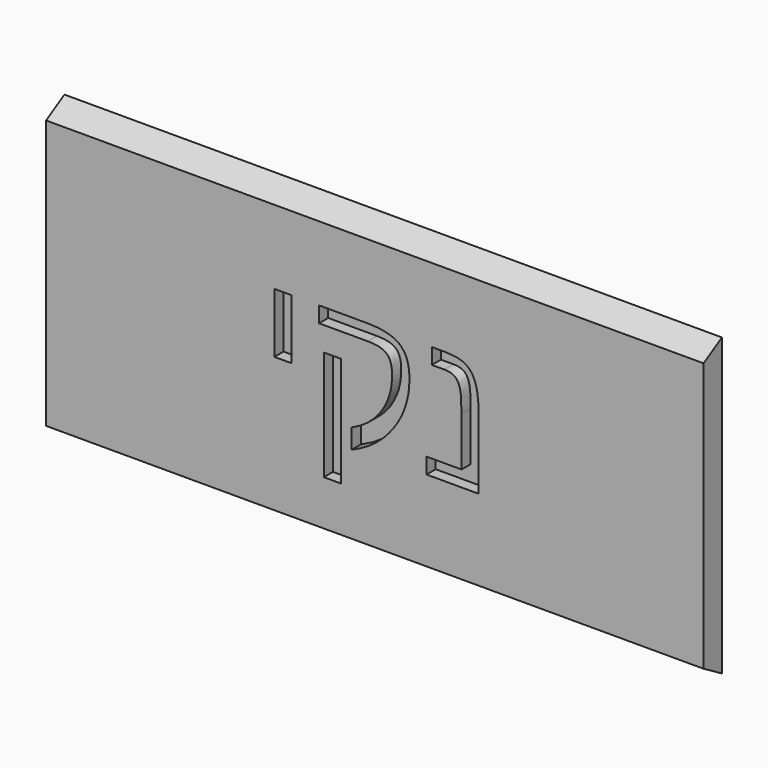
from build123d import *

# Parameters (mm, degrees)
F1_DEPTH     = 36
F2_TEXT_SIZE = 20.8333333333
F3_DEPTH     = 1.3


# Not quite as in the source:
# - Text() gives the source's letters only with a copy of the font that has no kerning and outlines rounded to 1/6400 em; it was checked with that copy


with BuildPart() as f1:
    # F0 (on Right) → F1 (new body, symmetric)
    with BuildSketch(Plane.YZ):
        Polygon((1.2569191167, -16.1964185536), (1.257158001, 16.1968544126), (-1.2568556704, 14.7234033793), (-1.2568556704, -14.7232851014), align=None)
    extrude(amount=F1_DEPTH, both=True)

    # F2 (on Front) → F3 (cut)
    with BuildSketch(Plane.XZ):
        with Locations((-12.7726552787, -5.8618432602)):
            Text('יקנ', F2_TEXT_SIZE, font='Arimo', text_align=(TextAlign.LEFT, TextAlign.BOTTOM))
    extrude(amount=F3_DEPTH, mode=Mode.SUBTRACT)


solid = f1.part
